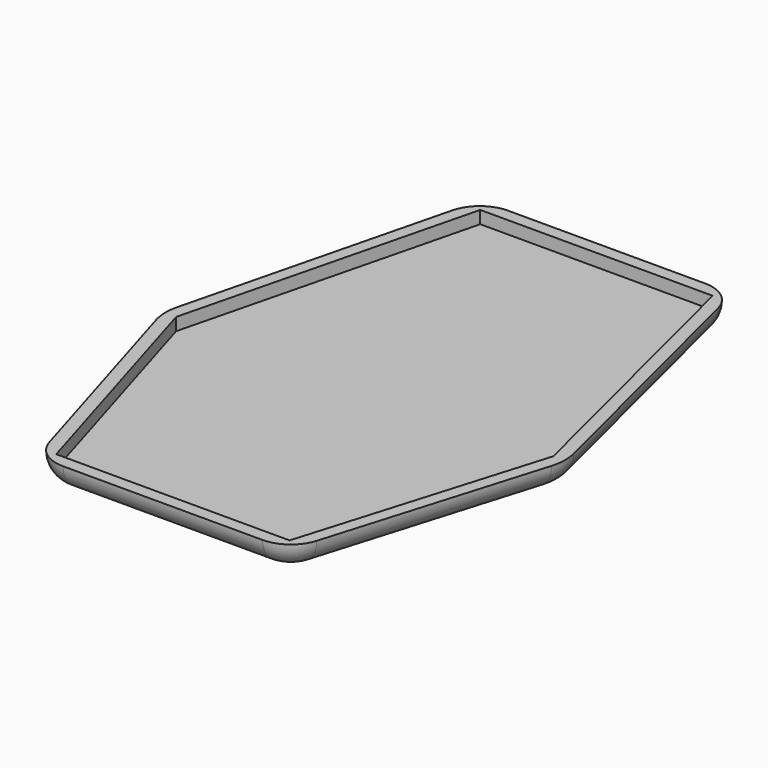
from build123d import *

# Parameters (mm, degrees)
F1_DEPTH = 5
F2_T     = -2.5
F3_R     = 7
F4_R     = 7
F5_R     = 10
F6_R     = 10
F7_R     = 7
F8_R     = 7
F9_R     = 4.99999


# Not quite as in the source:
# - a fillet or chamfer is up to 0.001 mm smaller than in the source, because OpenCascade refuses the exact size


with BuildPart() as f1:
    # F0 (on Top) → F1 (new body)
    with BuildSketch(Plane.XY):
        Polygon((25, 55), (-25, 55), (-40, -5), (-25, -55), (25, -55), (40, -5), align=None)
    extrude(amount=F1_DEPTH)

    # F2
    f2_openings = [f1.faces().sort_by_distance(p)[0] for p in [
        (0, -0.384615, 5),
    ]]
    offset(amount=F2_T, openings=f2_openings)

    # F3
    f3_edges = [f1.edges().sort_by_distance(p)[0] for p in [
        (25, 55, 2.5),
    ]]
    fillet(f3_edges, radius=F3_R)

    # F4
    f4_edges = [f1.edges().sort_by_distance(p)[0] for p in [
        (-25, 55, 2.5),
    ]]
    fillet(f4_edges, radius=F4_R)

    # F5
    f5_edges = [f1.edges().sort_by_distance(p)[0] for p in [
        (-40, -5, 2.5),
    ]]
    fillet(f5_edges, radius=F5_R)

    # F6
    f6_edges = [f1.edges().sort_by_distance(p)[0] for p in [
        (40, -5, 2.5),
    ]]
    fillet(f6_edges, radius=F6_R)

    # F7
    f7_edges = [f1.edges().sort_by_distance(p)[0] for p in [
        (-25, -55, 2.5),
    ]]
    fillet(f7_edges, radius=F7_R)

    # F8
    f8_edges = [f1.edges().sort_by_distance(p)[0] for p in [
        (25, -55, 2.5),
    ]]
    fillet(f8_edges, radius=F8_R)

    # F9 (radius 5 in the source; OpenCascade refuses exactly that, so slightly less here)
    f9_edges = [f1.edges().sort_by_distance(p)[0] for p in [
        (32.853411, -28.821964, 0),
    ]]
    fillet(f9_edges, radius=F9_R)


solid = f1.part
